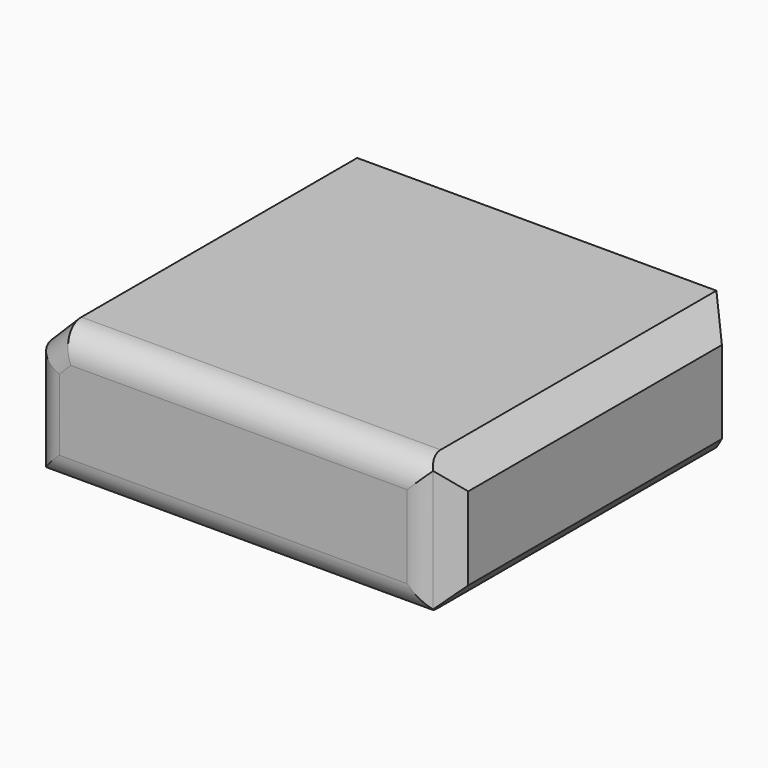
from build123d import *

# Parameters (mm, degrees)
F0_W        = 76.2943662703
F0_H        = 68.5328170657
F1_DEPTH    = 25.4
F2_SIZE     = 5.08
F3_T1_DEPTH = 45.72
F3_T3_DEPTH = 32.5842048969
F3_T5_DEPTH = 96.6143662703
F3_T7_DEPTH = 91.5343662703
F3_T9_DEPTH = 35.9210244843


# Not quite as in the source:
# - a fillet or chamfer that OpenCascade refuses, or shapes differently, is made with other operations: its cross-section is extruded or revolved along the edge and cut away or added


with BuildPart() as f1:
    # F0 (on Top) → F1 (new body)
    with BuildSketch(Plane.XY):
        with Locations((-1.9816737622, 2.3119486868)):
            Rectangle(F0_W, F0_H)
    extrude(amount=F1_DEPTH)

    # F2
    f2_edges = [f1.edges().sort_by_distance(p)[0] for p in [
        (36.165509, -31.95446, 12.7),
        (36.165509, 36.578357, 12.7),
        (36.165509, 2.311949, 0),
        (36.165509, 2.311949, 25.4),
        (-40.128857, 2.311949, 25.4),
    ]]
    chamfer(f2_edges, length=F2_SIZE)

    # F3: fillet of radius 5.08 on 5 edges, made by hand

    # F3_s2 → F3_t1 (cut)
    with BuildSketch(Plane.XY.offset(-12.7)):
        with BuildLine():
            ThreePointArc((-40.1288568974, -26.874459846), (-38.6409593458, -30.4665622944), (-35.0488568974, -31.954459846))
            Line((-35.0488568974, -31.954459846), (-40.1288568974, -31.954459846))
            Line((-40.1288568974, -31.954459846), (-40.1288568974, -26.874459846))
        make_face()
    extrude(amount=F3_T1_DEPTH, mode=Mode.SUBTRACT)

    # F3_s4 → F3_t3 (cut)
    with BuildSketch(Plane(origin=(-18.8846845697, 0, -18.8846845697), x_dir=(0, 1, 0), z_dir=(0.7071067812, 0, 0.7071067812))):
        with BuildLine():
            ThreePointArc((-26.874459846, 42.7437966271), (-30.4665622944, 41.2558990755), (-31.954459846, 37.6637966271))
            Line((-31.954459846, 37.6637966271), (-31.954459846, 42.7437966271))
            Line((-31.954459846, 42.7437966271), (-26.874459846, 42.7437966271))
        make_face()
    extrude(amount=F3_T3_DEPTH, mode=Mode.SUBTRACT)

    # F3_s6 → F3_t5 (cut)
    with BuildSketch(Plane.YZ.offset(-52.8288568974)):
        with BuildLine():
            ThreePointArc((-26.874459846, 0), (-30.4665622944, 1.4878975516), (-31.954459846, 5.08))
            Line((-31.954459846, 5.08), (-31.954459846, 0))
            Line((-31.954459846, 0), (-26.874459846, 0))
        make_face()
    extrude(amount=F3_T5_DEPTH, mode=Mode.SUBTRACT)

    # F3_s8 → F3_t7 (cut)
    with BuildSketch(Plane.YZ.offset(-47.7488568974)):
        with BuildLine():
            ThreePointArc((-26.874459846, 25.4), (-30.4665622944, 23.9121024484), (-31.954459846, 20.32))
            Line((-31.954459846, 20.32), (-31.954459846, 25.4))
            Line((-31.954459846, 25.4), (-26.874459846, 25.4))
        make_face()
    extrude(amount=F3_T7_DEPTH, mode=Mode.SUBTRACT)

    # F3_s10 → F3_t9 (cut)
    with BuildSketch(Plane.XY.offset(-5.2605122421)):
        with BuildLine():
            ThreePointArc((28.9813044761, -31.954459846), (30.9253363125, -31.5677678712), (32.5734069245, -30.4665622944))
            Line((32.5734069245, -30.4665622944), (31.0855093729, -31.954459846))
            Line((31.0855093729, -31.954459846), (28.9813044761, -31.954459846))
        make_face()
    extrude(amount=F3_T9_DEPTH, mode=Mode.SUBTRACT)


solid = f1.part
